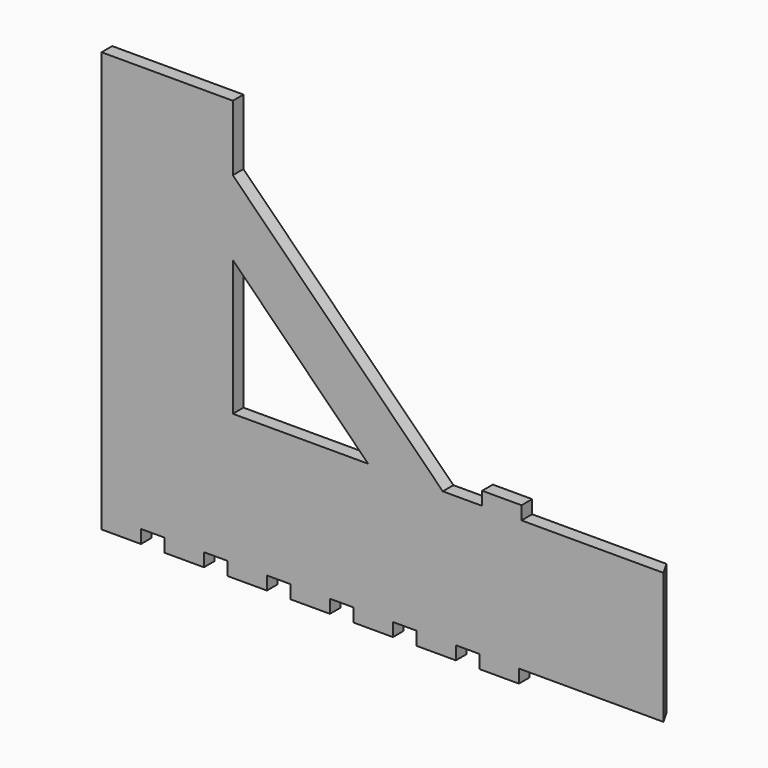
from build123d import *

# Parameters (mm, degrees)
F0_W     = 15
F0_H     = 5.08
F1_DEPTH = 5.08
F2_DEPTH = 25
F4_DEPTH = 58
F5_W     = 15
F5_H     = 5.08
F6_DEPTH = 5.08


# Not quite as in the source:
# - a feature names something its author has since deleted; it is built from what else it names


with BuildPart() as f1:
    # F0 (on Front) → F1 (new body)
    with BuildSketch(Plane.XZ):
        Polygon((-87.5, 0), (-32.419, 0), (-32.419, 50), (-116.5, 50), (-144.9023774395, 50), (-196.5, 50), (-196.5, 101.5976225605), (-196.5, 130), (-246.5, 130), (-246.5, 0), (-231.5, 0), (-222.5, 0), (-207.5, 0), (-198.5, 0), (-183.5, 0), (-174.5, 0), (-159.5, 0), (-150.5, 0), (-135.5, 0), (-126.5, 0), (-111.5, 0), (-102.5, 0), align=None)
        with Locations((-95, -2.54)):
            Rectangle(F0_W, F0_H)
        Polygon((-144.9023774395, 50), (-116.5, 50), (-196.5, 130), (-196.5, 101.5976225605), align=None)
        with Locations((-119, -2.54)):
            Rectangle(F0_W, F0_H)
        with Locations((-143, -2.54)):
            Rectangle(F0_W, F0_H)
        with Locations((-239, -2.54)):
            Rectangle(F0_W, F0_H)
        with Locations((-167, -2.54)):
            Rectangle(F0_W, F0_H)
        with Locations((-215, -2.54)):
            Rectangle(F0_W, F0_H)
        with Locations((-191, -2.54)):
            Rectangle(F0_W, F0_H)
    extrude(amount=F1_DEPTH)

    # F2 (add): a face of the model
    f2_faces = [f1.faces().sort_by_distance(p)[0] for p in [
        (-221.5, -2.54, 130),
    ]]
    extrude(f2_faces, amount=F2_DEPTH)

    # F3 (on face) → F4 (cut)
    with BuildSketch(Plane(origin=(0, 0, 0), x_dir=(1, 0, 0), z_dir=(0, 0, -1))):
        Polygon((-32.419, 0), (-32.419, 5.08), (-35.3519393675, 0), align=None)
    extrude(amount=-F4_DEPTH, mode=Mode.SUBTRACT)

    # F5 (on face) → F6 (join)
    with BuildSketch(Plane.XY.offset(50)):
        with Locations((-94, -2.54)):
            Rectangle(F5_W, F5_H)
    extrude(amount=F6_DEPTH)


solid = f1.part
